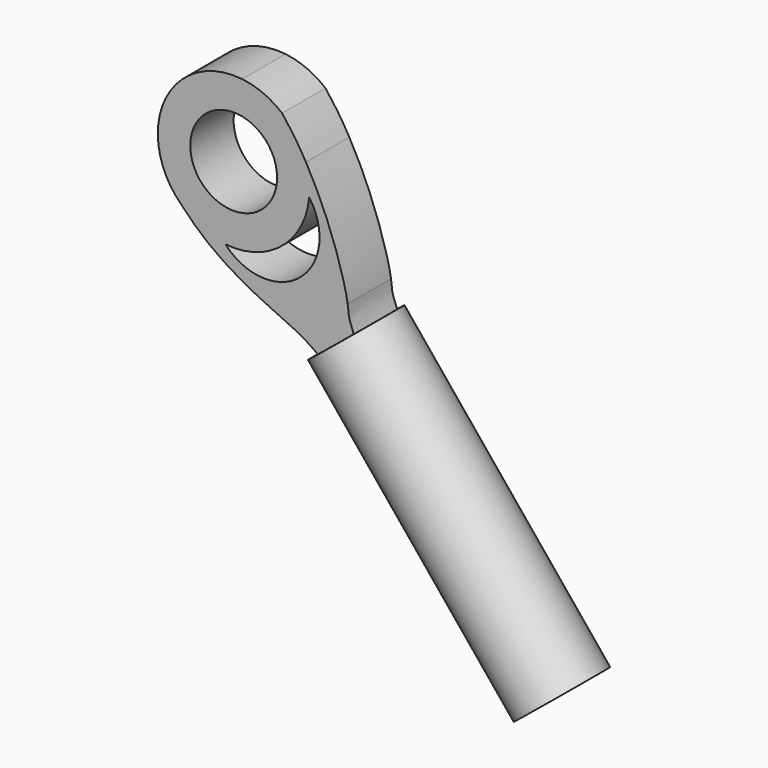
from build123d import *

# Parameters (mm, degrees)
F1_R     = 5.084021356
F2_DEPTH = 6.35
F3_R     = 5.08
F4_DEPTH = 38.1


with BuildPart() as f2:
    # F1 (on face) → F2 (new body)
    with BuildSketch(Plane.XZ):
        with BuildLine():
            ThreePointArc((-23.435486266, -2.0356566424), (-23.4073623703, -1.6282166531), (-23.3979811386, -1.2199149375))
            ThreePointArc((-23.3979811386, -1.2199149375), (-23.502785805, 0.1411298632), (-23.8147287088, 1.4700838098))
            add(Edge.make_bspline(
                [(-26.6112679949, 5.621651249), (-25.5726723735, 4.3377625486), (-24.6409406575, 2.9236120143), (-23.8147287088, 1.4700838098)],
                knots=[0, 0, 0, 0, 0.1448384022, 0.1448384022, 0.1448384022, 0.1448384022], degree=3))
            ThreePointArc((-26.6112679949, 5.621651249), (-28.8068112918, 6.9601557527), (-31.2935971509, 7.6142969959))
            Line((-31.2935971509, 7.6142969959), (-23.6553535863, -1.7499138663))
            ThreePointArc((-23.6553535863, -1.7499138663), (-23.5433915196, -1.8912244789), (-23.435486266, -2.0356566424))
        make_face()
        with BuildLine():
            ThreePointArc((-23.8147287088, 1.4700838098), (-23.502785805, 0.1411298632), (-23.3979811386, -1.2199149375))
            ThreePointArc((-23.3979811386, -1.2199149375), (-23.4073623703, -1.6282166531), (-23.435486266, -2.0356566424))
            ThreePointArc((-23.435486266, -2.0356566424), (-24.5585613429, -10.6811993954), (-33.2543862597, -10.0572313368))
            ThreePointArc((-33.2543862597, -10.0572313368), (-36.0145517074, -9.2911460577), (-38.3878110502, -7.6870762197))
            add(Edge.make_bspline(
                [(-38.3878110502, -7.6870762197), (-33.7082410797, -12.8874080847), (-27.843105649, -14.8041480157), (-24.8275432116, -16.3721035764)],
                knots=[0, 0, 0, 0, 0.6549803292, 0.6549803292, 0.6549803292, 0.6549803292], degree=3))
            Line((-24.8275432116, -16.3721035764), (-18.9267995353, -11.5507319804))
            add(Edge.make_bspline(
                [(-23.8147287088, 1.4700838098), (-20.8244478634, -3.7906214549), (-19.2163795919, -9.5671382328), (-18.9267995353, -11.5507319804)],
                knots=[0.1448384022, 0.1448384022, 0.1448384022, 0.1448384022, 0.6690471122, 0.6690471122, 0.6690471122, 0.6690471122], degree=3))
        make_face()
        with BuildLine():
            ThreePointArc((-33.2543862597, -10.0572313368), (-26.6635684549, -8.1045414316), (-23.435486266, -2.0356566424))
            ThreePointArc((-23.435486266, -2.0356566424), (-23.5433915196, -1.8912244789), (-23.6553535863, -1.7499138663))
            Line((-23.6553535863, -1.7499138663), (-31.2935971509, 7.6142969959))
            ThreePointArc((-31.2935971509, 7.6142969959), (-37.9022105078, 5.6730182981), (-41.1406471645, -0.4060327385))
            Line((-41.1406471645, -0.4060327385), (-33.4966443619, -9.7773042187))
            ThreePointArc((-33.4966443619, -9.7773042187), (-33.3775556867, -9.9190335859), (-33.2543862597, -10.0572313368))
        make_face()
        with Locations((-32.2879811386, -1.2199149375)):
            Circle(F1_R, mode=Mode.SUBTRACT)
        with BuildLine():
            add(Edge.make_bspline(
                [(-18.9267995353, -11.5507319804), (-18.7439766364, -12.8030501249), (-19.0866869126, -12.5435558307), (-17.5587098689, -15.9462096301)],
                knots=[0.6690471122, 0.6690471122, 0.6690471122, 0.6690471122, 1, 1, 1, 1], degree=3))
            Line((-18.9267995353, -11.5507319804), (-24.8275432116, -16.3721035764))
            add(Edge.make_bspline(
                [(-24.8275432116, -16.3721035764), (-23.2390552632, -17.1980451921), (-22.4412659418, -17.9272062293), (-21.1053046157, -18.8440564292)],
                knots=[0.6549803292, 0.6549803292, 0.6549803292, 0.6549803292, 1, 1, 1, 1], degree=3))
            Line((-21.1053046157, -18.8440564292), (-17.5587098689, -15.9462096301))
        make_face()
        with BuildLine():
            ThreePointArc((-38.3878110502, -7.6870762197), (-36.0145517074, -9.2911460577), (-33.2543862597, -10.0572313368))
            ThreePointArc((-33.2543862597, -10.0572313368), (-33.3775556867, -9.9190335859), (-33.4966443619, -9.7773042187))
            Line((-33.4966443619, -9.7773042187), (-41.1406471645, -0.4060327385))
            ThreePointArc((-41.1406471645, -0.4060327385), (-40.6034896759, -4.3638643274), (-38.3878110502, -7.6870762197))
        make_face()
        Polygon((5.5537237598, -44.232879484), (-17.5587098689, -15.9462096301), (-21.1053046157, -18.8440564292), (2.007129013, -47.1307262831), align=None)
    extrude(amount=F2_DEPTH)


with BuildPart() as f4:
    # F3 (on face) → F4 (new body)
    with BuildSketch(Plane(origin=(23.8960697274, 0, -29.2457404549), x_dir=(0.7743758105, 0, 0.6327259312), z_dir=(0.6327259312, 0, -0.7743758105))):
        with Locations((-26.0512717068, 3.2741681207)):
            Circle(F3_R)
        with BuildLine():
            ThreePointArc((-23.6866205246, 6.2615624345), (-22.6215908904, 4.9335021732), (-22.2412717068, 3.2741681207))
            ThreePointArc((-22.2412717068, 3.2741681207), (-22.6215908904, 1.6148340682), (-23.6866205246, 0.2867738069))
            Line((-23.6866205246, 0.2867738069), (-23.6866205246, 0))
            Line((-23.6866205246, 0), (-24.1029588168, 0))
            ThreePointArc((-24.1029588168, 0), (-26.0512717068, -0.5358318793), (-27.9995845968, 0))
            Line((-27.9995845968, 0), (-28.2665605208, 0))
            Line((-28.2665605208, 0), (-28.2665605208, 0.174394666))
            ThreePointArc((-28.2665605208, 0.174394666), (-29.139118789, 5.506050823), (-23.8028593224, 6.35))
            Line((-23.8028593224, 6.35), (-23.6866205246, 6.35))
            Line((-23.6866205246, 6.35), (-23.6866205246, 6.2615624345))
        make_face(mode=Mode.SUBTRACT)
    extrude(amount=-F4_DEPTH)


solid = Compound([f2.part, f4.part])
